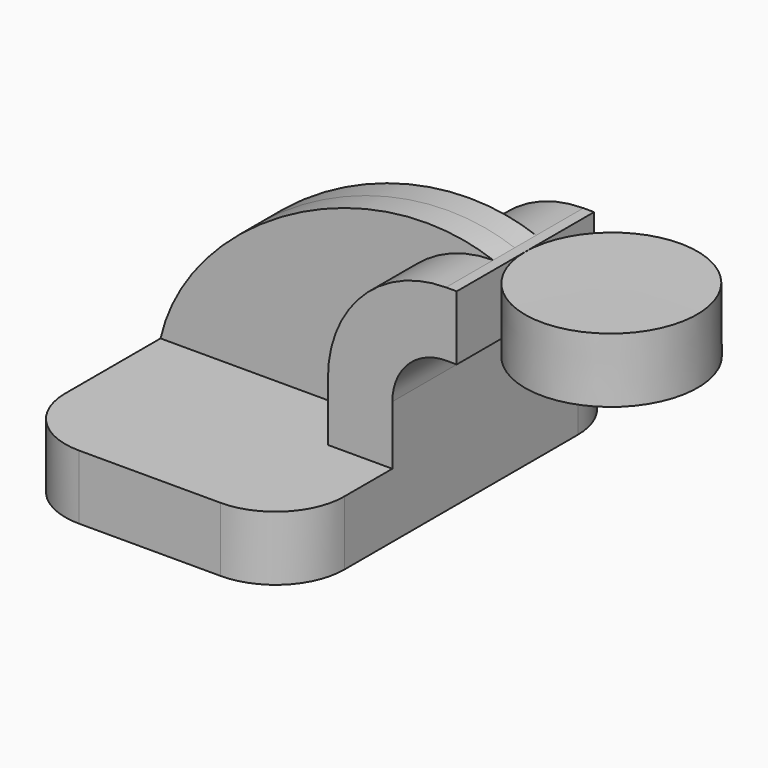
from build123d import *

# Parameters (mm, degrees)
F1_DEPTH = 63.5
F2_DEPTH = 25.4
F3_DEPTH = 7.9375
F5_R     = 20.32


# Not quite as in the source:
# - a feature names something its author has since deleted; it is built from what else it names


with BuildPart() as f1:
    # F0 (on Front) → F1 (new body, symmetric)
    with BuildSketch(Plane.XZ):
        Polygon((22.225, 9.525), (-41.275, 9.525), (-41.275, -9.525), (41.275, -9.525), (41.275, 9.525), align=None)
    extrude(amount=F1_DEPTH, both=True)

    # F0 (on Front) → F2 (join, symmetric)
    with BuildSketch(Plane.XZ):
        with BuildLine():
            Line((22.225, 27.0002), (22.225, 9.525))
            Line((22.225, 9.525), (41.275, 9.525))
            Line((41.275, 9.525), (41.275, 27.0002))
            ThreePointArc((41.275, 27.0002), (45.9246798487, 38.2255201513), (57.15, 42.8752))
            Line((57.15, 42.8752), (60.325, 42.8752))
            Line((60.325, 42.8752), (60.325, 61.9252))
            Line((60.325, 61.9252), (57.15, 61.9252))
            ThreePointArc((57.15, 61.9252), (32.4542956671, 51.6959043329), (22.225, 27.0002))
        make_face()
    extrude(amount=F2_DEPTH, both=True)

    # F0 (on Front) → F3 (join, symmetric)
    with BuildSketch(Plane.XZ):
        with BuildLine():
            add(Edge.make_bspline(
                [(-41.275, 9.525), (-33.1754907966, 45.2206768095), (19.6965429932, 75.4829570651), (57.15, 61.9252)],
                knots=[0, 0, 0, 0, 111.5045361635, 111.5045361635, 111.5045361635, 111.5045361635], degree=3))
            Line((-41.275, 9.525), (22.225, 9.525))
            Line((22.225, 9.525), (22.225, 27.0002))
            ThreePointArc((22.225, 27.0002), (32.4542956671, 51.6959043329), (57.15, 61.9252))
        make_face()
    extrude(amount=F3_DEPTH, both=True)

    # F0 (on Front) → F4 (revolve)
    with BuildSketch(Plane.XZ):
        Polygon((85.7438487918, 61.9252), (60.325, 61.9252), (60.325, 42.8752), (85.8194455504, 42.8752), align=None)
    revolve(axis=Axis((85.7816471711, 0, 52.4002), (0.0039683025, 0, -0.9999921263)))

    # F5
    f5_edges = [f1.edges().sort_by_distance(p)[0] for p in [
        (41.275, 63.5, 0),
        (-41.275, 63.5, 0),
        (-41.275, -63.5, 0),
        (41.275, -63.5, 0),
    ]]
    fillet(f5_edges, radius=F5_R)


solid = f1.part
